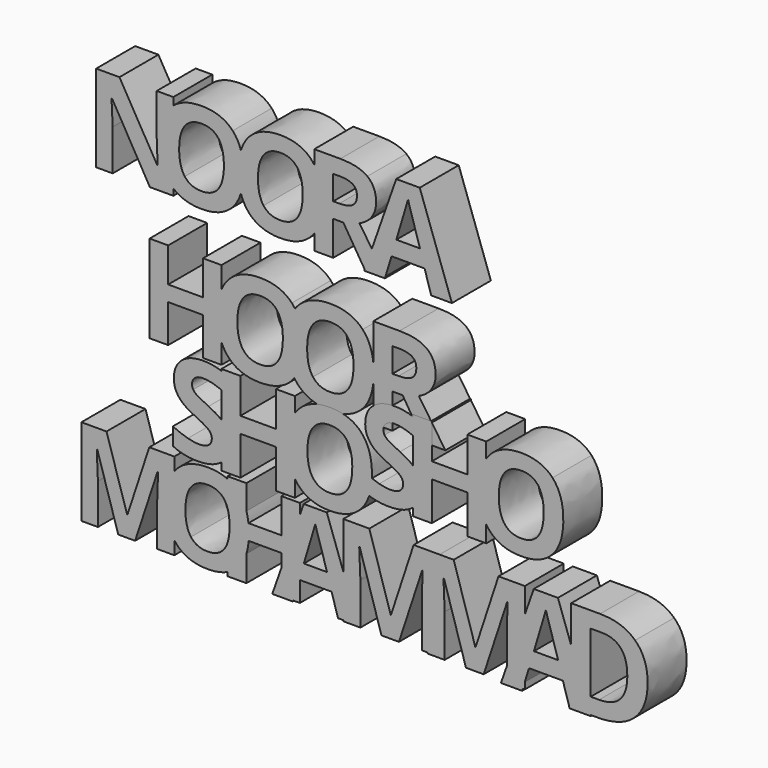
from build123d import *

# Parameters (mm, degrees)
F4_DEPTH = 25
F5_DEPTH = 25
F6_DEPTH = 25
F2_W     = 6.2625637302
F2_H     = 46.2371155878


with BuildPart() as f4:
    # F0 (on Front) → F4 (new body)
    with BuildSketch(Plane.XZ):
        with BuildLine():
            Line((-21.3353137972, -33.1943402998), (-11.8071950997, -33.1943402998))
            Line((-11.8071950997, -33.1943402998), (-11.8071950997, -23.0057868832))
            add(Edge.make_bspline(
                [(-11.8071950997, -23.0057868832), (-13.9013277173, -17.99866493), (-13.9013277173, -11.0128203345)],
                knots=[0.3919372789, 0.3919372789, 0.3919372789, 1, 1, 1], degree=2))
            add(Edge.make_bspline(
                [(-13.9013277173, -11.0128203345), (-13.9013277173, -4.036271611), (-11.8071950997, 0.9371130219)],
                knots=[0, 0, 0, 0.6072535887, 0.6072535887, 0.6072535887], degree=2))
            Line((-11.8071950997, 0.9371130219), (-11.8071950997, 11.8718857132))
            Line((-11.8071950997, 11.8718857132), (-21.3353137972, 11.8718857132))
            Line((-21.3353137972, 11.8718857132), (-21.3353137972, -5.793601437))
            Line((-21.3353137972, -5.793601437), (-39.1783435318, -5.793601437))
            Line((-39.1783435318, -5.793601437), (-39.1783435318, 11.8718857132))
            Line((-39.1783435318, 11.8718857132), (-48.73605266, 11.8718857132))
            Line((-48.73605266, 11.8718857132), (-48.73605266, -33.1943402998))
            Line((-48.73605266, -33.1943402998), (-39.1783435318, -33.1943402998))
            Line((-39.1783435318, -33.1943402998), (-39.1783435318, -13.7435638284))
            Line((-39.1783435318, -13.7435638284), (-21.3353137972, -13.7435638284))
            Line((-21.3353137972, -13.7435638284), (-21.3353137972, -33.1943402998))
        make_face()
        with BuildLine():
            add(Edge.make_bspline(
                [(-11.8071950997, -23.0057868832), (-13.9013277173, -17.99866493), (-13.9013277173, -11.0128203345)],
                knots=[0.3919372789, 0.3919372789, 0.3919372789, 1, 1, 1], degree=2))
            Line((-11.8071950997, -23.0057868832), (-11.8071950997, 0.9371130219))
            add(Edge.make_bspline(
                [(-13.9013277173, -11.0128203345), (-13.9013277173, -4.036271611), (-11.8071950997, 0.9371130219)],
                knots=[0, 0, 0, 0.6072535887, 0.6072535887, 0.6072535887], degree=2))
        make_face()
        with BuildLine():
            Line((-11.8071950997, 0.9371130219), (-11.8071950997, -23.0057868832))
            add(Edge.make_bspline(
                [(-8.237534045, -28.6385462427), (-10.457385925, -26.2332134056), (-11.8071950997, -23.0057868832)],
                knots=[0, 0, 0, 0.3919372789, 0.3919372789, 0.3919372789], degree=2))
            add(Edge.make_bspline(
                [(7.9986744822, -34.7755813418), (-2.5737403727, -34.7755813418), (-8.237534045, -28.6385462427)],
                knots=[0, 0, 0, 1, 1, 1], degree=2))
            add(Edge.make_bspline(
                [(24.2348830094, -28.6385462427), (18.5710893372, -34.7755813418), (7.9986744822, -34.7755813418)],
                knots=[0, 0, 0, 1, 1, 1], degree=2))
            add(Edge.make_bspline(
                [(25.5832055823, -26.9929228199), (24.9547978497, -27.858478518), (24.2348830094, -28.6385462427)],
                knots=[0.8728917609, 0.8728917609, 0.8728917609, 1, 1, 1], degree=2))
            add(Edge.make_bspline(
                [(25.5832055823, -26.9929228199), (21.7115614933, -21.0599088889), (21.7115614933, -11.4686214765)],
                knots=[0.1811928258, 0.1811928258, 0.1811928258, 1, 1, 1], degree=2))
            add(Edge.make_bspline(
                [(21.7115614933, -11.4686214765), (21.7115614933, -1.5095593905), (25.8969432134, 4.4459327701)],
                knots=[0, 0, 0, 0.8502040585, 0.8502040585, 0.8502040585], degree=2))
            add(Edge.make_bspline(
                [(24.2801933588, 6.4820090087), (25.1569815466, 5.5290125286), (25.8969432134, 4.4459327701)],
                knots=[0, 0, 0, 0.1560542476, 0.1560542476, 0.1560542476], degree=2))
            add(Edge.make_bspline(
                [(8.0590882814, 12.5888372083), (18.6617100359, 12.5888372083), (24.2801933588, 6.4820090087)],
                knots=[0, 0, 0, 1, 1, 1], degree=2))
            add(Edge.make_bspline(
                [(-8.2224305952, 6.5323538414), (-2.5435334731, 12.5888372083), (8.0590882814, 12.5888372083)],
                knots=[0, 0, 0, 1, 1, 1], degree=2))
            add(Edge.make_bspline(
                [(-11.8071950997, 0.9371130219), (-10.4527970599, 4.1536917341), (-8.2224305952, 6.5323538414)],
                knots=[0.6072535887, 0.6072535887, 0.6072535887, 1, 1, 1], degree=2))
        make_face()
        with BuildLine():
            add(Edge.make_bspline(
                [(-3.6712577243, -11.0732341337), (-3.6712577243, -18.7860624946), (-0.7462229478, -22.6877870243)],
                knots=[0, 0, 0, 1, 1, 1], degree=2))
            add(Edge.make_bspline(
                [(-0.7160160482, 0.5463532402), (-3.6712577243, -3.3704747394), (-3.6712577243, -11.0732341337)],
                knots=[0, 0, 0, 1, 1, 1], degree=2))
            add(Edge.make_bspline(
                [(8.0590882814, 4.4631812198), (2.2392256279, 4.4631812198), (-0.7160160482, 0.5463532402)],
                knots=[0, 0, 0, 1, 1, 1], degree=2))
            add(Edge.make_bspline(
                [(19.6686066888, -11.0732341337), (19.6686066888, 4.4631812198), (8.0590882814, 4.4631812198)],
                knots=[0, 0, 0, 1, 1, 1], degree=2))
            add(Edge.make_bspline(
                [(7.9986744822, -26.5895115541), (19.6686066888, -26.5895115541), (19.6686066888, -11.0732341337)],
                knots=[0, 0, 0, 1, 1, 1], degree=2))
            add(Edge.make_bspline(
                [(-0.7462229478, -22.6877870243), (2.1788118287, -26.5895115541), (7.9986744822, -26.5895115541)],
                knots=[0, 0, 0, 1, 1, 1], degree=2))
        make_face(mode=Mode.SUBTRACT)
        with BuildLine():
            add(Edge.make_bspline(
                [(25.5832055823, -26.9929228199), (21.7115614933, -21.0599088889), (21.7115614933, -11.4686214765)],
                knots=[0.1811928258, 0.1811928258, 0.1811928258, 1, 1, 1], degree=2))
            add(Edge.make_bspline(
                [(29.8986766817, -11.0732341337), (29.8986766817, -21.048882977), (25.5832055823, -26.9929228199)],
                knots=[0, 0, 0, 0.8728917609, 0.8728917609, 0.8728917609], degree=2))
            add(Edge.make_bspline(
                [(25.8969432134, 4.4459327701), (29.8986766817, -1.4113929713), (29.8986766817, -11.0732341337)],
                knots=[0.1560542476, 0.1560542476, 0.1560542476, 1, 1, 1], degree=2))
            add(Edge.make_bspline(
                [(21.7115614933, -11.4686214765), (21.7115614933, -1.5095593905), (25.8969432134, 4.4459327701)],
                knots=[0, 0, 0, 0.8502040585, 0.8502040585, 0.8502040585], degree=2))
        make_face()
        with BuildLine():
            add(Edge.make_bspline(
                [(29.8986766817, -11.0732341337), (29.8986766817, -21.048882977), (25.5832055823, -26.9929228199)],
                knots=[0, 0, 0, 0.8728917609, 0.8728917609, 0.8728917609], degree=2))
            add(Edge.make_bspline(
                [(27.4862976764, -29.4396004781), (26.4399569092, -28.3058321268), (25.5832055823, -26.9929228199)],
                knots=[0, 0, 0, 0.1811928258, 0.1811928258, 0.1811928258], degree=2))
            add(Edge.make_bspline(
                [(44.0405414011, -35.6968479511), (33.2610338594, -35.6968479511), (27.4862976764, -29.4396004781)],
                knots=[0, 0, 0, 1, 1, 1], degree=2))
            add(Edge.make_bspline(
                [(60.5947851258, -29.4396004781), (54.8200489428, -35.6968479511), (44.0405414011, -35.6968479511)],
                knots=[0, 0, 0, 1, 1, 1], degree=2))
            add(Edge.make_bspline(
                [(66.087589583, -16.4160509741), (65.0935584026, -24.5649297009), (60.5947851258, -29.4396004781)],
                knots=[0.2209560516, 0.2209560516, 0.2209560516, 1, 1, 1], degree=2))
            Line((66.087589583, -16.4160509741), (66.087589583, -6.6192053935))
            add(Edge.make_bspline(
                [(60.6409830153, 6.3688969555), (65.0986725029, 1.5237559622), (66.087589583, -6.6192053935)],
                knots=[0, 0, 0, 0.7781547856, 0.7781547856, 0.7781547856], degree=2))
            add(Edge.make_bspline(
                [(44.102138587, 12.5953458356), (54.9124447217, 12.5953458356), (60.6409830153, 6.3688969555)],
                knots=[0, 0, 0, 1, 1, 1], degree=2))
            add(Edge.make_bspline(
                [(27.5016969728, 6.4202279438), (33.2918324524, 12.5953458356), (44.102138587, 12.5953458356)],
                knots=[0, 0, 0, 1, 1, 1], degree=2))
            add(Edge.make_bspline(
                [(25.8969432134, 4.4459327701), (26.6343581774, 5.4952203455), (27.5016969728, 6.4202279438)],
                knots=[0.8502040585, 0.8502040585, 0.8502040585, 1, 1, 1], degree=2))
            add(Edge.make_bspline(
                [(25.8969432134, 4.4459327701), (29.8986766817, -1.4113929713), (29.8986766817, -11.0732341337)],
                knots=[0.1560542476, 0.1560542476, 0.1560542476, 1, 1, 1], degree=2))
        make_face()
        with BuildLine():
            add(Edge.make_bspline(
                [(32.1420183146, -11.5302186625), (32.1420183146, -19.3941260691), (35.1243487345, -23.3722776618)],
                knots=[0, 0, 0, 1, 1, 1], degree=2))
            add(Edge.make_bspline(
                [(35.1551473274, 0.3169734357), (32.1420183146, -3.6765774535), (32.1420183146, -11.5302186625)],
                knots=[0, 0, 0, 1, 1, 1], degree=2))
            add(Edge.make_bspline(
                [(44.102138587, 4.310524325), (38.1682763403, 4.310524325), (35.1551473274, 0.3169734357)],
                knots=[0, 0, 0, 1, 1, 1], degree=2))
            add(Edge.make_bspline(
                [(55.9390644876, -11.5302186625), (55.9390644876, 4.310524325), (44.102138587, 4.310524325)],
                knots=[0, 0, 0, 1, 1, 1], degree=2))
            add(Edge.make_bspline(
                [(44.0405414011, -27.3504292546), (55.9390644876, -27.3504292546), (55.9390644876, -11.5302186625)],
                knots=[0, 0, 0, 1, 1, 1], degree=2))
            add(Edge.make_bspline(
                [(35.1243487345, -23.3722776618), (38.1066791543, -27.3504292546), (44.0405414011, -27.3504292546)],
                knots=[0, 0, 0, 1, 1, 1], degree=2))
        make_face(mode=Mode.SUBTRACT)
        with BuildLine():
            Line((66.087589583, -6.6192053935), (66.087589583, -16.4160509741))
            add(Edge.make_bspline(
                [(66.3695213088, -11.5302186625), (66.3695213088, -14.10482826), (66.087589583, -16.4160509741)],
                knots=[0, 0, 0, 0.2209560516, 0.2209560516, 0.2209560516], degree=2))
            add(Edge.make_bspline(
                [(66.087589583, -6.6192053935), (66.3695213088, -8.9406934074), (66.3695213088, -11.5302186625)],
                knots=[0.7781547856, 0.7781547856, 0.7781547856, 1, 1, 1], degree=2))
        make_face()
        with BuildLine():
            add(Edge.make_bspline(
                [(66.3695213088, -11.5302186625), (66.3695213088, -14.10482826), (66.087589583, -16.4160509741)],
                knots=[0, 0, 0, 0.2209560516, 0.2209560516, 0.2209560516], degree=2))
            Line((66.087589583, -16.4160509741), (66.087589583, -34.4568653964))
            Line((66.087589583, -34.4568653964), (75.9107906423, -34.4568653964))
            Line((75.9107906423, -34.4568653964), (75.9107906423, -16.6858938206))
            Line((75.9107906423, -16.6858938206), (81.131583775, -16.6858938206))
            Line((81.131583775, -16.6858938206), (92.1915552462, -34.4568653964))
            Line((92.1915552462, -34.4568653964), (103.0893273192, -34.4568653964))
            add(Edge.make_bspline(
                [(89.4645778624, -14.2731777709), (99.9264390525, -29.8950073193), (103.0893273192, -34.4568653964)],
                knots=[0, 0, 0, 1, 1, 1], degree=2))
            add(Edge.make_bspline(
                [(95.8359729767, -9.2855462733), (93.5905250565, -12.4687094649), (89.4645778624, -14.2731777709)],
                knots=[0, 0, 0, 1, 1, 1], degree=2))
            add(Edge.make_bspline(
                [(98.0814208969, -2.0169857372), (98.0814208969, -6.1023830818), (95.8359729767, -9.2855462733)],
                knots=[0, 0, 0, 1, 1, 1], degree=2))
            add(Edge.make_bspline(
                [(93.5550439382, 8.4246005281), (98.0814208969, 4.9880007767), (98.0814208969, -2.0169857372)],
                knots=[0, 0, 0, 1, 1, 1], degree=2))
            add(Edge.make_bspline(
                [(79.5805520288, 11.8612002795), (89.0286669795, 11.8612002795), (93.5550439382, 8.4246005281)],
                knots=[0, 0, 0, 1, 1, 1], degree=2))
            Line((79.5805520288, 11.8612002795), (66.087589583, 11.8612002795))
            Line((66.087589583, 11.8612002795), (66.087589583, -6.6192053935))
            add(Edge.make_bspline(
                [(66.087589583, -6.6192053935), (66.3695213088, -8.9406934074), (66.3695213088, -11.5302186625)],
                knots=[0.7781547856, 0.7781547856, 0.7781547856, 1, 1, 1], degree=2))
        make_face()
        with BuildLine():
            Line((79.0736789091, -8.6975734545), (75.9107906423, -8.6975734545))
            Line((75.9107906423, -8.6975734545), (75.9107906423, 3.8120551391))
            Line((75.9107906423, 3.8120551391), (78.891204586, 3.8120551391))
            add(Edge.make_bspline(
                [(85.9012598311, 2.4181540599), (83.6355369861, 3.8120551391), (78.891204586, 3.8120551391)],
                knots=[0, 0, 0, 1, 1, 1], degree=2))
            add(Edge.make_bspline(
                [(88.166982676, -2.270422297), (88.166982676, 1.0242529808), (85.9012598311, 2.4181540599)],
                knots=[0, 0, 0, 1, 1, 1], degree=2))
            add(Edge.make_bspline(
                [(85.9519471431, -7.1465417083), (88.166982676, -5.5955099621), (88.166982676, -2.270422297)],
                knots=[0, 0, 0, 1, 1, 1], degree=2))
            add(Edge.make_bspline(
                [(79.0736789091, -8.6975734545), (83.7369116101, -8.6975734545), (85.9519471431, -7.1465417083)],
                knots=[0, 0, 0, 1, 1, 1], degree=2))
        make_face(mode=Mode.SUBTRACT)
    extrude(amount=F4_DEPTH)


with BuildPart() as f5:
    # F1 (on Front) → F5 (new body)
    with BuildSketch(Plane.XZ):
        with BuildLine():
            Line((-48.5764728851, 35.1428589012), (-36.5549885101, 35.1428589012))
            Line((-36.5549885101, 35.1428589012), (-36.5549885101, 38.4932039616))
            add(Edge.make_bspline(
                [(-36.5549885101, 38.4932039616), (-37.337133854, 39.1602999713), (-38.0419799443, 39.9240398682)],
                knots=[0.8734596848, 0.8734596848, 0.8734596848, 1, 1, 1], degree=2))
            add(Edge.make_bspline(
                [(-38.0419799443, 39.9240398682), (-43.6121106118, 45.9595858982), (-43.6121106118, 57.2582865055)],
                knots=[0, 0, 0, 1, 1, 1], degree=2))
            add(Edge.make_bspline(
                [(-43.6121106118, 57.2582865055), (-43.6121106118, 68.5569871128), (-38.0271262626, 74.5133135066)],
                knots=[0, 0, 0, 1, 1, 1], degree=2))
            add(Edge.make_bspline(
                [(-38.0271262626, 74.5133135066), (-37.328899138, 75.257965307), (-36.5549885101, 75.9095217551)],
                knots=[0, 0, 0, 0.1250186358, 0.1250186358, 0.1250186358], degree=2))
            Line((-36.5549885101, 75.9095217551), (-36.5549885101, 79.7619995262))
            Line((-36.5549885101, 79.7619995262), (-45.0706135101, 79.7619995262))
            Line((-45.0706135101, 79.7619995262), (-45.0706135101, 58.6389526512))
            add(Edge.make_bspline(
                [(-44.6116291351, 46.3440307762), (-45.0706135101, 55.0452026512), (-45.0706135101, 58.6389526512)],
                knots=[0, 0, 0, 1, 1, 1], degree=2))
            Line((-44.6116291351, 46.3440307762), (-44.8264728851, 46.3440307762))
            Line((-44.8264728851, 46.3440307762), (-64.2014728851, 79.7619995262))
            Line((-64.2014728851, 79.7619995262), (-76.1350666351, 79.7619995262))
            Line((-76.1350666351, 79.7619995262), (-76.1350666351, 35.1428589012))
            Line((-76.1350666351, 35.1428589012), (-67.6780353851, 35.1428589012))
            Line((-67.6780353851, 35.1428589012), (-67.6780353851, 56.1389526512))
            add(Edge.make_bspline(
                [(-68.2639728851, 68.8928589012), (-67.6780353851, 59.9573120262), (-67.6780353851, 56.1389526512)],
                knots=[0, 0, 0, 1, 1, 1], degree=2))
            Line((-68.2639728851, 68.8928589012), (-67.9905353851, 68.8928589012))
            Line((-67.9905353851, 68.8928589012), (-48.5764728851, 35.1428589012))
        make_face()
        with BuildLine():
            add(Edge.make_bspline(
                [(-36.5549885101, 38.4932039616), (-37.337133854, 39.1602999713), (-38.0419799443, 39.9240398682)],
                knots=[0.8734596848, 0.8734596848, 0.8734596848, 1, 1, 1], degree=2))
            Line((-36.5549885101, 38.4932039616), (-36.5549885101, 75.9095217551))
            add(Edge.make_bspline(
                [(-38.0271262626, 74.5133135066), (-37.328899138, 75.257965307), (-36.5549885101, 75.9095217551)],
                knots=[0, 0, 0, 0.1250186358, 0.1250186358, 0.1250186358], degree=2))
            add(Edge.make_bspline(
                [(-43.6121106118, 57.2582865055), (-43.6121106118, 68.5569871128), (-38.0271262626, 74.5133135066)],
                knots=[0, 0, 0, 1, 1, 1], degree=2))
            add(Edge.make_bspline(
                [(-38.0419799443, 39.9240398682), (-43.6121106118, 45.9595858982), (-43.6121106118, 57.2582865055)],
                knots=[0, 0, 0, 1, 1, 1], degree=2))
        make_face()
        with BuildLine():
            Line((-36.5549885101, 75.9095217551), (-36.5549885101, 38.4932039616))
            add(Edge.make_bspline(
                [(-22.0742720308, 33.8884938383), (-31.1561365749, 33.8884938383), (-36.5549885101, 38.4932039616)],
                knots=[0, 0, 0, 0.8734596848, 0.8734596848, 0.8734596848], degree=2))
            add(Edge.make_bspline(
                [(-6.1065641174, 39.9240398682), (-11.6766947848, 33.8884938383), (-22.0742720308, 33.8884938383)],
                knots=[0, 0, 0, 1, 1, 1], degree=2))
            add(Edge.make_bspline(
                [(-1.8486114519, 47.5145455032), (-3.2399502207, 43.0301752816), (-6.1065641174, 39.9240398682)],
                knots=[0.4853596679, 0.4853596679, 0.4853596679, 1, 1, 1], degree=2))
            add(Edge.make_bspline(
                [(-1.8486114519, 47.5145455032), (-3.1656606093, 51.7641834469), (-3.1656606093, 57.2582865055)],
                knots=[0.5137402743, 0.5137402743, 0.5137402743, 1, 1, 1], degree=2))
            add(Edge.make_bspline(
                [(-3.1656606093, 57.2582865055), (-3.1656606093, 62.729767225), (-1.8559519315, 66.94843264)],
                knots=[0, 0, 0, 0.4842575186, 0.4842575186, 0.4842575186], degree=2))
            add(Edge.make_bspline(
                [(-6.062003072, 74.463801234), (-3.2366355234, 71.3928596243), (-1.8559519315, 66.94843264)],
                knots=[0, 0, 0, 0.5113260246, 0.5113260246, 0.5113260246], degree=2))
            add(Edge.make_bspline(
                [(-22.0148573037, 80.4696399004), (-11.5875726942, 80.4696399004), (-6.062003072, 74.463801234)],
                knots=[0, 0, 0, 1, 1, 1], degree=2))
            add(Edge.make_bspline(
                [(-36.5549885101, 75.9095217551), (-31.1385370158, 80.4696399004), (-22.0148573037, 80.4696399004)],
                knots=[0.1250186358, 0.1250186358, 0.1250186358, 1, 1, 1], degree=2))
        make_face()
        with BuildLine():
            add(Edge.make_bspline(
                [(-33.5512168195, 57.1988717784), (-33.5512168195, 49.6135916161), (-30.6745537815, 45.7763904896)],
                knots=[0, 0, 0, 1, 1, 1], degree=2))
            add(Edge.make_bspline(
                [(-30.6448464179, 68.6263042945), (-33.5512168195, 64.7742494862), (-33.5512168195, 57.1988717784)],
                knots=[0, 0, 0, 1, 1, 1], degree=2))
            add(Edge.make_bspline(
                [(-22.0148573037, 72.4783591027), (-27.7384760163, 72.4783591027), (-30.6448464179, 68.6263042945)],
                knots=[0, 0, 0, 1, 1, 1], degree=2))
            add(Edge.make_bspline(
                [(-10.5973272422, 57.1988717784), (-10.5973272422, 72.4783591027), (-22.0148573037, 72.4783591027)],
                knots=[0, 0, 0, 1, 1, 1], degree=2))
            add(Edge.make_bspline(
                [(-22.0742720308, 41.9391893631), (-10.5973272422, 41.9391893631), (-10.5973272422, 57.1988717784)],
                knots=[0, 0, 0, 1, 1, 1], degree=2))
            add(Edge.make_bspline(
                [(-30.6745537815, 45.7763904896), (-27.7978907434, 41.9391893631), (-22.0742720308, 41.9391893631)],
                knots=[0, 0, 0, 1, 1, 1], degree=2))
        make_face(mode=Mode.SUBTRACT)
        with BuildLine():
            add(Edge.make_bspline(
                [(-1.8486114519, 47.5145455032), (-3.1656606093, 51.7641834469), (-3.1656606093, 57.2582865055)],
                knots=[0.5137402743, 0.5137402743, 0.5137402743, 1, 1, 1], degree=2))
            add(Edge.make_bspline(
                [(-0.5364334499, 57.1988717784), (-0.5364334499, 51.7437757163), (-1.8486114519, 47.5145455032)],
                knots=[0, 0, 0, 0.4853596679, 0.4853596679, 0.4853596679], degree=2))
            add(Edge.make_bspline(
                [(-1.8559519315, 66.94843264), (-0.5364334499, 62.7008964337), (-0.5364334499, 57.1988717784)],
                knots=[0.5113260246, 0.5113260246, 0.5113260246, 1, 1, 1], degree=2))
            add(Edge.make_bspline(
                [(-3.1656606093, 57.2582865055), (-3.1656606093, 62.729767225), (-1.8559519315, 66.94843264)],
                knots=[0, 0, 0, 0.4842575186, 0.4842575186, 0.4842575186], degree=2))
        make_face()
        with BuildLine():
            add(Edge.make_bspline(
                [(-0.5364334499, 57.1988717784), (-0.5364334499, 51.7437757163), (-1.8486114519, 47.5145455032)],
                knots=[0, 0, 0, 0.4853596679, 0.4853596679, 0.4853596679], degree=2))
            add(Edge.make_bspline(
                [(2.4044700582, 39.9240398682), (-0.4571303986, 43.0247429409), (-1.8486114519, 47.5145455032)],
                knots=[0, 0, 0, 0.5137402743, 0.5137402743, 0.5137402743], degree=2))
            add(Edge.make_bspline(
                [(18.3721779716, 33.8884938383), (7.9746007256, 33.8884938383), (2.4044700582, 39.9240398682)],
                knots=[0, 0, 0, 1, 1, 1], degree=2))
            add(Edge.make_bspline(
                [(34.3398858851, 39.9240398682), (28.7697552176, 33.8884938383), (18.3721779716, 33.8884938383)],
                knots=[0, 0, 0, 1, 1, 1], degree=2))
            add(Edge.make_bspline(
                [(35.7973932629, 41.7259413865), (35.1238020662, 40.7734566014), (34.3398858851, 39.9240398682)],
                knots=[0.8592643103, 0.8592643103, 0.8592643103, 1, 1, 1], degree=2))
            Line((35.7973932629, 41.7259413865), (35.7973932629, 72.7158650742))
            add(Edge.make_bspline(
                [(34.3844469305, 74.463801234), (35.1429853678, 73.6393324845), (35.7973932629, 72.7158650742)],
                knots=[0, 0, 0, 0.1372778716, 0.1372778716, 0.1372778716], degree=2))
            add(Edge.make_bspline(
                [(18.4315926988, 80.4696399004), (28.8588773083, 80.4696399004), (34.3844469305, 74.463801234)],
                knots=[0, 0, 0, 1, 1, 1], degree=2))
            add(Edge.make_bspline(
                [(2.4193237399, 74.5133135066), (8.0043080892, 80.4696399004), (18.4315926988, 80.4696399004)],
                knots=[0, 0, 0, 1, 1, 1], degree=2))
            add(Edge.make_bspline(
                [(-1.8559519315, 66.94843264), (-0.461089947, 71.4413829522), (2.4193237399, 74.5133135066)],
                knots=[0.4842575186, 0.4842575186, 0.4842575186, 1, 1, 1], degree=2))
            add(Edge.make_bspline(
                [(-1.8559519315, 66.94843264), (-0.5364334499, 62.7008964337), (-0.5364334499, 57.1988717784)],
                knots=[0.5113260246, 0.5113260246, 0.5113260246, 1, 1, 1], degree=2))
        make_face()
        with BuildLine():
            add(Edge.make_bspline(
                [(6.895233183, 57.1988717784), (6.895233183, 49.6135916161), (9.771896221, 45.7763904896)],
                knots=[0, 0, 0, 1, 1, 1], degree=2))
            add(Edge.make_bspline(
                [(9.8016035846, 68.6263042945), (6.895233183, 64.7742494862), (6.895233183, 57.1988717784)],
                knots=[0, 0, 0, 1, 1, 1], degree=2))
            add(Edge.make_bspline(
                [(18.4315926988, 72.4783591027), (12.7079739862, 72.4783591027), (9.8016035846, 68.6263042945)],
                knots=[0, 0, 0, 1, 1, 1], degree=2))
            add(Edge.make_bspline(
                [(29.8491227603, 57.1988717784), (29.8491227603, 72.4783591027), (18.4315926988, 72.4783591027)],
                knots=[0, 0, 0, 1, 1, 1], degree=2))
            add(Edge.make_bspline(
                [(18.3721779716, 41.9391893631), (29.8491227603, 41.9391893631), (29.8491227603, 57.1988717784)],
                knots=[0, 0, 0, 1, 1, 1], degree=2))
            add(Edge.make_bspline(
                [(9.771896221, 45.7763904896), (12.6485592591, 41.9391893631), (18.3721779716, 41.9391893631)],
                knots=[0, 0, 0, 1, 1, 1], degree=2))
        make_face(mode=Mode.SUBTRACT)
        with BuildLine():
            Line((35.7973932629, 72.7158650742), (35.7973932629, 41.7259413865))
            add(Edge.make_bspline(
                [(39.9100165526, 57.1988717784), (39.9100165526, 47.541354548), (35.7973932629, 41.7259413865)],
                knots=[0, 0, 0, 0.8592643103, 0.8592643103, 0.8592643103], degree=2))
            add(Edge.make_bspline(
                [(35.7973932629, 72.7158650742), (39.9100165526, 66.9123385475), (39.9100165526, 57.1988717784)],
                knots=[0.1372778716, 0.1372778716, 0.1372778716, 1, 1, 1], degree=2))
        make_face()
        with BuildLine():
            add(Edge.make_bspline(
                [(39.9100165526, 57.1988717784), (39.9100165526, 47.541354548), (35.7973932629, 41.7259413865)],
                knots=[0, 0, 0, 0.8592643103, 0.8592643103, 0.8592643103], degree=2))
            Line((35.7973932629, 41.7259413865), (35.7973932629, 33.8131673634))
            Line((35.7973932629, 33.8131673634), (45.5399000121, 33.8131673634))
            Line((45.5399000121, 33.8131673634), (45.5399000121, 51.4381563534))
            Line((45.5399000121, 51.4381563534), (50.7178060759, 51.4381563534))
            Line((50.7178060759, 51.4381563534), (61.6644474176, 33.8492816769))
            Line((61.6644474176, 33.8492816769), (65.3522718239, 44.3388900938))
            add(Edge.make_bspline(
                [(58.9823474049, 53.8310527479), (62.6096596302, 48.4146882719), (65.3522718239, 44.3388900938)],
                knots=[0, 0, 0, 0.3495894388, 0.3495894388, 0.3495894388], degree=2))
            add(Edge.make_bspline(
                [(65.30140364, 58.7777125215), (63.0744013233, 55.6206979505), (58.9823474049, 53.8310527479)],
                knots=[0, 0, 0, 1, 1, 1], degree=2))
            add(Edge.make_bspline(
                [(67.5284059568, 65.9865642647), (67.5284059568, 61.9347270924), (65.30140364, 58.7777125215)],
                knots=[0, 0, 0, 1, 1, 1], degree=2))
            add(Edge.make_bspline(
                [(63.0392116704, 76.3423763923), (67.5284059568, 72.934007158), (67.5284059568, 65.9865642647)],
                knots=[0, 0, 0, 1, 1, 1], degree=2))
            add(Edge.make_bspline(
                [(49.1795155365, 79.7507456265), (58.550017384, 79.7507456265), (63.0392116704, 76.3423763923)],
                knots=[0, 0, 0, 1, 1, 1], degree=2))
            Line((49.1795155365, 79.7507456265), (35.7973932629, 79.7507456265))
            Line((35.7973932629, 79.7507456265), (35.7973932629, 72.7158650742))
            add(Edge.make_bspline(
                [(35.7973932629, 72.7158650742), (39.9100165526, 66.9123385475), (39.9100165526, 57.1988717784)],
                knots=[0.1372778716, 0.1372778716, 0.1372778716, 1, 1, 1], degree=2))
        make_face()
        with BuildLine():
            Line((48.6768062099, 59.3608553403), (45.5399000121, 59.3608553403))
            Line((45.5399000121, 59.3608553403), (45.5399000121, 71.7677215204))
            Line((45.5399000121, 71.7677215204), (48.4958308524, 71.7677215204))
            add(Edge.make_bspline(
                [(55.448300839, 70.3852708723), (53.2011901492, 71.7677215204), (48.4958308524, 71.7677215204)],
                knots=[0, 0, 0, 1, 1, 1], degree=2))
            add(Edge.make_bspline(
                [(57.6954115288, 65.7352096014), (57.6954115288, 69.0028202242), (55.448300839, 70.3852708723)],
                knots=[0, 0, 0, 1, 1, 1], degree=2))
            add(Edge.make_bspline(
                [(55.4985717717, 60.8991458796), (57.6954115288, 62.437436419), (57.6954115288, 65.7352096014)],
                knots=[0, 0, 0, 1, 1, 1], degree=2))
            add(Edge.make_bspline(
                [(48.6768062099, 59.3608553403), (53.3017320145, 59.3608553403), (55.4985717717, 60.8991458796)],
                knots=[0, 0, 0, 1, 1, 1], degree=2))
        make_face(mode=Mode.SUBTRACT)
        with BuildLine():
            Line((65.3522718239, 44.3388900938), (61.6644474176, 33.8492816769))
            Line((61.6644474176, 33.8492816769), (61.6869235819, 33.8131673634))
            Line((61.6869235819, 33.8131673634), (72.2655823064, 33.8131673634))
            Line((72.2655823064, 33.8131673634), (72.33566955, 34.0435447683))
            add(Edge.make_bspline(
                [(65.3522718239, 44.3388900938), (70.260972013, 37.0440668107), (72.33566955, 34.0435447683)],
                knots=[0.3495894388, 0.3495894388, 0.3495894388, 0.9752811602, 0.9752811602, 0.9752811602], degree=2))
        make_face()
        Polygon((61.6869235819, 33.8131673634), (61.6644474176, 33.8492816769), (61.421725899, 33.1588871777), (72.0665319926, 33.1588871777), (72.2655823064, 33.8131673634), align=None)
        with BuildLine():
            Line((77.8681552371, 79.9389354128), (65.3522718239, 44.3388900938))
            add(Edge.make_bspline(
                [(65.3522718239, 44.3388900938), (70.260972013, 37.0440668107), (72.33566955, 34.0435447683)],
                knots=[0.3495894388, 0.3495894388, 0.3495894388, 0.9752811602, 0.9752811602, 0.9752811602], degree=2))
            Line((72.33566955, 34.0435447683), (75.4414657253, 44.2523249458))
            Line((75.4414657253, 44.2523249458), (92.4282923077, 44.2523249458))
            Line((92.4282923077, 44.2523249458), (95.8032260404, 33.1588871777))
            Line((95.8032260404, 33.1588871777), (106.448032134, 33.1588871777))
            Line((106.448032134, 33.1588871777), (89.9404257494, 79.9389354128))
            Line((89.9404257494, 79.9389354128), (77.8681552371, 79.9389354128))
        make_face()
        with BuildLine():
            add(Edge.make_bspline(
                [(90.0627798424, 52.5316185741), (85.382735784, 67.6015643656), (84.7913576677, 69.579622203)],
                knots=[0, 0, 0, 1, 1, 1], degree=2))
            Line((90.0627798424, 52.5316185741), (77.9293322836, 52.5316185741))
            add(Edge.make_bspline(
                [(83.9450751909, 72.6996515752), (82.8948692257, 68.6211818076), (77.9293322836, 52.5316185741)],
                knots=[0, 0, 0, 1, 1, 1], degree=2))
            add(Edge.make_bspline(
                [(84.7913576677, 69.579622203), (84.1999795514, 71.5576800403), (83.9450751909, 72.6996515752)],
                knots=[0, 0, 0, 1, 1, 1], degree=2))
        make_face(mode=Mode.SUBTRACT)
        with BuildLine():
            Line((72.33566955, 34.0435447683), (72.2655823064, 33.8131673634))
            Line((72.2655823064, 33.8131673634), (72.4951741034, 33.8131673634))
            add(Edge.make_bspline(
                [(72.33566955, 34.0435447683), (72.4176334217, 33.925004885), (72.4951741034, 33.8131673634)],
                knots=[0.9752811602, 0.9752811602, 0.9752811602, 1, 1, 1], degree=2))
        make_face()
    extrude(amount=F5_DEPTH)


with BuildPart() as f6:
    # F3 (on Front) → F6 (new body)
    with BuildSketch(Plane.XZ):
        with BuildLine():
            add(Edge.make_bspline(
                [(-9.773376744, -60.1399672845), (-7.4308009773, -63.172986435), (-7.4308009773, -67.5819606149)],
                knots=[0, 0, 0, 1, 1, 1], degree=2))
            add(Edge.make_bspline(
                [(-7.4308009773, -67.5819606149), (-7.4308009773, -73.6874528237), (-11.8249799418, -77.203782343)],
                knots=[0, 0, 0, 1, 1, 1], degree=2))
            add(Edge.make_bspline(
                [(-11.8249799418, -77.203782343), (-11.8411305754, -77.2167064752), (-11.857327512, -77.2295831053)],
                knots=[0, 0, 0, 0.003675461, 0.003675461, 0.003675461], degree=2))
            Line((-11.857327512, -77.2295831053), (-11.857327512, -81.0456089675))
            Line((-11.857327512, -81.0456089675), (-2.1004989459, -81.0456089675))
            Line((-2.1004989459, -81.0456089675), (-2.1004989459, -61.1896069733))
            Line((-2.1004989459, -61.1896069733), (16.1142615042, -61.1896069733))
            Line((16.1142615042, -61.1896069733), (16.1142615042, -81.0456089675))
            Line((16.1142615042, -81.0456089675), (25.8408831707, -81.0456089675))
            Line((25.8408831707, -81.0456089675), (25.8408831707, -72.4579250864))
            add(Edge.make_bspline(
                [(25.8408831707, -72.4579250864), (22.1995292231, -66.7496005995), (22.1995292231, -57.600601227)],
                knots=[0.1926675383, 0.1926675383, 0.1926675383, 1, 1, 1], degree=2))
            add(Edge.make_bspline(
                [(22.1995292231, -57.600601227), (22.1995292231, -48.4637761771), (25.8408831707, -42.8101256923)],
                knots=[0, 0, 0, 0.8062581665, 0.8062581665, 0.8062581665], degree=2))
            Line((25.8408831707, -42.8101256923), (25.8408831707, -35.0405008988))
            Line((25.8408831707, -35.0405008988), (16.1142615042, -35.0405008988))
            Line((16.1142615042, -35.0405008988), (16.1142615042, -53.0740199514))
            Line((16.1142615042, -53.0740199514), (-2.1004989459, -53.0740199514))
            Line((-2.1004989459, -53.0740199514), (-2.1004989459, -35.0405008988))
            Line((-2.1004989459, -35.0405008988), (-11.857327512, -35.0405008988))
            Line((-11.857327512, -35.0405008988), (-11.857327512, -35.9465561363))
            add(Edge.make_bspline(
                [(-11.857327512, -35.9465561363), (-9.8085950891, -36.6209872168), (-7.6477974694, -37.5575368934)],
                knots=[0.3794034527, 0.3794034527, 0.3794034527, 1, 1, 1], degree=2))
            Line((-7.6477974694, -37.5575368934), (-10.7252022661, -44.9945984854))
            add(Edge.make_bspline(
                [(-10.7252022661, -44.9945984854), (-11.3075641299, -44.7559255904), (-11.857327512, -44.5404823221)],
                knots=[0, 0, 0, 0.1613176213, 0.1613176213, 0.1613176213], degree=2))
            Line((-11.857327512, -44.5404823221), (-11.857327512, -58.0527789062))
            add(Edge.make_bspline(
                [(-11.857327512, -58.0527789062), (-10.5796303791, -59.096080999), (-9.773376744, -60.1399672845)],
                knots=[0.6558260157, 0.6558260157, 0.6558260157, 1, 1, 1], degree=2))
        make_face()
        with BuildLine():
            add(Edge.make_bspline(
                [(-7.4308009773, -67.5819606149), (-7.4308009773, -73.6874528237), (-11.8249799418, -77.203782343)],
                knots=[0, 0, 0, 1, 1, 1], degree=2))
            add(Edge.make_bspline(
                [(-9.773376744, -60.1399672845), (-7.4308009773, -63.172986435), (-7.4308009773, -67.5819606149)],
                knots=[0, 0, 0, 1, 1, 1], degree=2))
            add(Edge.make_bspline(
                [(-11.857327512, -58.0527789062), (-10.5796303791, -59.096080999), (-9.773376744, -60.1399672845)],
                knots=[0.6558260157, 0.6558260157, 0.6558260157, 1, 1, 1], degree=2))
            Line((-11.857327512, -58.0527789062), (-11.857327512, -77.2295831053))
            add(Edge.make_bspline(
                [(-11.8249799418, -77.203782343), (-11.8411305754, -77.2167064752), (-11.857327512, -77.2295831053)],
                knots=[0, 0, 0, 0.003675461, 0.003675461, 0.003675461], degree=2))
        make_face()
        with BuildLine():
            add(Edge.make_bspline(
                [(-11.857327512, -77.2295831053), (-16.2479073967, -80.7201118623), (-24.0408960979, -80.7201118623)],
                knots=[0.003675461, 0.003675461, 0.003675461, 1, 1, 1], degree=2))
            Line((-11.857327512, -77.2295831053), (-11.857327512, -58.0527789062))
            add(Edge.make_bspline(
                [(-18.4384412116, -54.0788607218), (-14.2919886375, -56.0647592245), (-11.857327512, -58.0527789062)],
                knots=[0, 0, 0, 0.6558260157, 0.6558260157, 0.6558260157], degree=2))
            add(Edge.make_bspline(
                [(-24.4896842974, -50.9225481098), (-23.2123640372, -51.800397555), (-18.4384412116, -54.0788607218)],
                knots=[0, 0, 0, 1, 1, 1], degree=2))
            add(Edge.make_bspline(
                [(-26.3538814339, -49.1027366194), (-25.7670045576, -50.0446986646), (-24.4896842974, -50.9225481098)],
                knots=[0, 0, 0, 1, 1, 1], degree=2))
            add(Edge.make_bspline(
                [(-26.9407583101, -46.8982495295), (-26.9407583101, -48.1607745743), (-26.3538814339, -49.1027366194)],
                knots=[0, 0, 0, 1, 1, 1], degree=2))
            add(Edge.make_bspline(
                [(-25.490827204, -43.6038482407), (-26.9407583101, -44.8663732855), (-26.9407583101, -46.8982495295)],
                knots=[0, 0, 0, 1, 1, 1], degree=2))
            add(Edge.make_bspline(
                [(-21.328439947, -42.3413231959), (-24.0408960979, -42.3413231959), (-25.490827204, -43.6038482407)],
                knots=[0, 0, 0, 1, 1, 1], degree=2))
            add(Edge.make_bspline(
                [(-16.6926057981, -42.9282000722), (-19.0499767802, -42.3413231959), (-21.328439947, -42.3413231959)],
                knots=[0, 0, 0, 1, 1, 1], degree=2))
            add(Edge.make_bspline(
                [(-11.857327512, -44.5404823221), (-14.7155202954, -43.4204033668), (-16.6926057981, -42.9282000722)],
                knots=[0.1613176213, 0.1613176213, 0.1613176213, 1, 1, 1], degree=2))
            Line((-11.857327512, -44.5404823221), (-11.857327512, -35.9465561363))
            add(Edge.make_bspline(
                [(-14.3204396006, -35.2198928651), (-13.1098258676, -35.5342407896), (-11.857327512, -35.9465561363)],
                knots=[0, 0, 0, 0.3794034527, 0.3794034527, 0.3794034527], degree=2))
            add(Edge.make_bspline(
                [(-21.0226721627, -34.3913608045), (-17.5112743818, -34.3913608045), (-14.3204396006, -35.2198928651)],
                knots=[0, 0, 0, 1, 1, 1], degree=2))
            add(Edge.make_bspline(
                [(-32.2275819352, -37.8090555546), (-28.1736929242, -34.3913608045), (-21.0226721627, -34.3913608045)],
                knots=[0, 0, 0, 1, 1, 1], degree=2))
            add(Edge.make_bspline(
                [(-36.2814709463, -47.2138807907), (-36.2814709463, -41.2267503048), (-32.2275819352, -37.8090555546)],
                knots=[0, 0, 0, 1, 1, 1], degree=2))
            add(Edge.make_bspline(
                [(-35.0485363322, -52.7571548155), (-36.2814709463, -50.3800568796), (-36.2814709463, -47.2138807907)],
                knots=[0, 0, 0, 1, 1, 1], degree=2))
            add(Edge.make_bspline(
                [(-31.749203305, -56.9195420725), (-33.8156017181, -55.1342527514), (-35.0485363322, -52.7571548155)],
                knots=[0, 0, 0, 1, 1, 1], degree=2))
            add(Edge.make_bspline(
                [(-25.5598715424, -60.6479363455), (-29.6828048918, -58.7048313937), (-31.749203305, -56.9195420725)],
                knots=[0, 0, 0, 1, 1, 1], degree=2))
            add(Edge.make_bspline(
                [(-19.7157614718, -63.7006824499), (-21.1508973625, -62.7488569278), (-25.5598715424, -60.6479363455)],
                knots=[0, 0, 0, 1, 1, 1], degree=2))
            add(Edge.make_bspline(
                [(-17.5408648126, -65.6881730477), (-18.280625581, -64.6525079719), (-19.7157614718, -63.7006824499)],
                knots=[0, 0, 0, 1, 1, 1], degree=2))
            add(Edge.make_bspline(
                [(-16.8011040441, -68.0455440298), (-16.8011040441, -66.7238381235), (-17.5408648126, -65.6881730477)],
                knots=[0, 0, 0, 1, 1, 1], degree=2))
            add(Edge.make_bspline(
                [(-18.4828268577, -71.6210544106), (-16.8011040441, -70.4226419657), (-16.8011040441, -68.0455440298)],
                knots=[0, 0, 0, 1, 1, 1], degree=2))
            add(Edge.make_bspline(
                [(-23.3011353294, -72.8194668554), (-20.1645496713, -72.8194668554), (-18.4828268577, -71.6210544106)],
                knots=[0, 0, 0, 1, 1, 1], degree=2))
            add(Edge.make_bspline(
                [(-29.0860645386, -71.9909347948), (-25.9248201882, -72.8194668554), (-23.3011353294, -72.8194668554)],
                knots=[0, 0, 0, 1, 1, 1], degree=2))
            add(Edge.make_bspline(
                [(-36.8042352226, -69.1206630133), (-32.2473088891, -71.1624027341), (-29.0860645386, -71.9909347948)],
                knots=[0, 0, 0, 1, 1, 1], degree=2))
            Line((-36.8042352226, -69.1206630133), (-36.8042352226, -77.9977922345))
            add(Edge.make_bspline(
                [(-24.0408960979, -80.7201118623), (-31.2609611978, -80.7201118623), (-36.8042352226, -77.9977922345)],
                knots=[0, 0, 0, 1, 1, 1], degree=2))
        make_face()
        with BuildLine():
            Line((-11.857327512, -35.9465561363), (-11.857327512, -44.5404823221))
            add(Edge.make_bspline(
                [(-10.7252022661, -44.9945984854), (-11.3075641299, -44.7559255904), (-11.857327512, -44.5404823221)],
                knots=[0, 0, 0, 0.1613176213, 0.1613176213, 0.1613176213], degree=2))
            Line((-10.7252022661, -44.9945984854), (-7.6477974694, -37.5575368934))
            add(Edge.make_bspline(
                [(-11.857327512, -35.9465561363), (-9.8085950891, -36.6209872168), (-7.6477974694, -37.5575368934)],
                knots=[0.3794034527, 0.3794034527, 0.3794034527, 1, 1, 1], degree=2))
        make_face()
        with BuildLine():
            add(Edge.make_bspline(
                [(25.8408831707, -72.4579250864), (22.1995292231, -66.7496005995), (22.1995292231, -57.600601227)],
                knots=[0.1926675383, 0.1926675383, 0.1926675383, 1, 1, 1], degree=2))
            Line((25.8408831707, -72.4579250864), (25.8408831707, -42.8101256923))
            add(Edge.make_bspline(
                [(22.1995292231, -57.600601227), (22.1995292231, -48.4637761771), (25.8408831707, -42.8101256923)],
                knots=[0, 0, 0, 0.8062581665, 0.8062581665, 0.8062581665], degree=2))
        make_face()
        with BuildLine():
            Line((25.8408831707, -42.8101256923), (25.8408831707, -72.4579250864))
            add(Edge.make_bspline(
                [(27.7862641378, -74.9865202815), (26.7098816745, -73.8202000835), (25.8408831707, -72.4579250864)],
                knots=[0, 0, 0, 0.1926675383, 0.1926675383, 0.1926675383], degree=2))
            add(Edge.make_bspline(
                [(43.8015708933, -81.0400579358), (33.3729990525, -81.0400579358), (27.7862641378, -74.9865202815)],
                knots=[0, 0, 0, 1, 1, 1], degree=2))
            add(Edge.make_bspline(
                [(59.8168776487, -74.9865202815), (54.230142734, -81.0400579358), (43.8015708933, -81.0400579358)],
                knots=[0, 0, 0, 1, 1, 1], degree=2))
            add(Edge.make_bspline(
                [(63.9854978765, -67.6943049535), (62.5888957332, -71.982884686), (59.8168776487, -74.9865202815)],
                knots=[0.5038214401, 0.5038214401, 0.5038214401, 1, 1, 1], degree=2))
            add(Edge.make_bspline(
                [(63.9854978765, -67.6943049535), (62.6635387575, -67.2220253013), (61.4252531353, -66.6138992662)],
                knots=[0.7766147557, 0.7766147557, 0.7766147557, 1, 1, 1], degree=2))
            Line((61.4252531353, -66.6138992662), (61.4252531353, -57.736770045))
            add(Edge.make_bspline(
                [(61.4252531353, -57.736770045), (63.5492553917, -58.6884333936), (65.3700414458, -59.3765236477)],
                knots=[0, 0, 0, 0.4661041458, 0.4661041458, 0.4661041458], degree=2))
            add(Edge.make_bspline(
                [(65.4036125634, -57.6601930661), (65.4036125634, -58.5340397989), (65.3700414458, -59.3765236477)],
                knots=[0, 0, 0, 0.0775182334, 0.0775182334, 0.0775182334], degree=2))
            add(Edge.make_bspline(
                [(59.861571528, -40.3437978239), (65.4036125634, -46.3675395586), (65.4036125634, -57.6601930661)],
                knots=[0, 0, 0, 1, 1, 1], degree=2))
            add(Edge.make_bspline(
                [(43.8611627324, -34.3200560892), (54.3195304926, -34.3200560892), (59.861571528, -40.3437978239)],
                knots=[0, 0, 0, 1, 1, 1], degree=2))
            add(Edge.make_bspline(
                [(27.8011620976, -40.294137958), (33.4027949721, -34.3200560892), (43.8611627324, -34.3200560892)],
                knots=[0, 0, 0, 1, 1, 1], degree=2))
            add(Edge.make_bspline(
                [(25.8408831707, -42.8101256923), (26.7158914739, -41.4515675327), (27.8011620976, -40.294137958)],
                knots=[0.8062581665, 0.8062581665, 0.8062581665, 1, 1, 1], degree=2))
        make_face()
        with BuildLine():
            add(Edge.make_bspline(
                [(32.2904139757, -57.6601930661), (32.2904139757, -65.2680845233), (35.175652185, -69.1167241312)],
                knots=[0, 0, 0, 1, 1, 1], degree=2))
            add(Edge.make_bspline(
                [(35.2054481045, -46.1986960145), (32.2904139757, -50.0622335821), (32.2904139757, -57.6601930661)],
                knots=[0, 0, 0, 1, 1, 1], degree=2))
            add(Edge.make_bspline(
                [(43.8611627324, -42.3351584468), (38.1204822334, -42.3351584468), (35.2054481045, -46.1986960145)],
                knots=[0, 0, 0, 1, 1, 1], degree=2))
            add(Edge.make_bspline(
                [(55.3127278108, -57.6601930661), (55.3127278108, -42.3351584468), (43.8611627324, -42.3351584468)],
                knots=[0, 0, 0, 1, 1, 1], degree=2))
            add(Edge.make_bspline(
                [(43.8015708933, -72.9653637391), (55.3127278108, -72.9653637391), (55.3127278108, -57.6601930661)],
                knots=[0, 0, 0, 1, 1, 1], degree=2))
            add(Edge.make_bspline(
                [(35.175652185, -69.1167241312), (38.0608903943, -72.9653637391), (43.8015708933, -72.9653637391)],
                knots=[0, 0, 0, 1, 1, 1], degree=2))
        make_face(mode=Mode.SUBTRACT)
        with BuildLine():
            add(Edge.make_bspline(
                [(63.9854978765, -67.6943049535), (62.6635387575, -67.2220253013), (61.4252531353, -66.6138992662)],
                knots=[0.7766147557, 0.7766147557, 0.7766147557, 1, 1, 1], degree=2))
            add(Edge.make_bspline(
                [(65.3700414458, -59.3765236477), (65.185420687, -64.0096731701), (63.9854978765, -67.6943049535)],
                knots=[0.0775182334, 0.0775182334, 0.0775182334, 0.5038214401, 0.5038214401, 0.5038214401], degree=2))
            add(Edge.make_bspline(
                [(61.4252531353, -57.736770045), (63.5492553917, -58.6884333936), (65.3700414458, -59.3765236477)],
                knots=[0, 0, 0, 0.4661041458, 0.4661041458, 0.4661041458], degree=2))
            Line((61.4252531353, -57.736770045), (61.4252531353, -66.6138992662))
        make_face()
        with BuildLine():
            add(Edge.make_bspline(
                [(65.3700414458, -59.3765236477), (65.185420687, -64.0096731701), (63.9854978765, -67.6943049535)],
                knots=[0.0775182334, 0.0775182334, 0.0775182334, 0.5038214401, 0.5038214401, 0.5038214401], degree=2))
            add(Edge.make_bspline(
                [(74.18859226, -69.336218894), (68.5813831663, -69.336218894), (63.9854978765, -67.6943049535)],
                knots=[0, 0, 0, 0.7766147557, 0.7766147557, 0.7766147557], degree=2))
            add(Edge.make_bspline(
                [(86.3721608459, -65.845690137), (81.9815809612, -69.336218894), (74.18859226, -69.336218894)],
                knots=[0.003675461, 0.003675461, 0.003675461, 1, 1, 1], degree=2))
            Line((86.3721608459, -65.845690137), (86.3721608459, -46.6688859379))
            add(Edge.make_bspline(
                [(79.7910471463, -42.6949677535), (83.9374997204, -44.6808662562), (86.3721608459, -46.6688859379)],
                knots=[0, 0, 0, 0.6558260157, 0.6558260157, 0.6558260157], degree=2))
            add(Edge.make_bspline(
                [(73.7398040605, -39.5386551415), (75.0171243207, -40.4165045867), (79.7910471463, -42.6949677535)],
                knots=[0, 0, 0, 1, 1, 1], degree=2))
            add(Edge.make_bspline(
                [(71.875606924, -37.7188436511), (72.4624838003, -38.6608056963), (73.7398040605, -39.5386551415)],
                knots=[0, 0, 0, 1, 1, 1], degree=2))
            add(Edge.make_bspline(
                [(71.2887300478, -35.5143565612), (71.2887300478, -36.776881606), (71.875606924, -37.7188436511)],
                knots=[0, 0, 0, 1, 1, 1], degree=2))
            add(Edge.make_bspline(
                [(72.7386611539, -32.2199552724), (71.2887300478, -33.4824803172), (71.2887300478, -35.5143565612)],
                knots=[0, 0, 0, 1, 1, 1], degree=2))
            add(Edge.make_bspline(
                [(76.9010484109, -30.9574302276), (74.18859226, -30.9574302276), (72.7386611539, -32.2199552724)],
                knots=[0, 0, 0, 1, 1, 1], degree=2))
            add(Edge.make_bspline(
                [(81.5368825598, -31.5443071039), (79.1795115777, -30.9574302276), (76.9010484109, -30.9574302276)],
                knots=[0, 0, 0, 1, 1, 1], degree=2))
            add(Edge.make_bspline(
                [(86.3721608459, -33.1565893538), (83.5139680625, -32.0365103985), (81.5368825598, -31.5443071039)],
                knots=[0.1613176213, 0.1613176213, 0.1613176213, 1, 1, 1], degree=2))
            Line((86.3721608459, -33.1565893538), (86.3721608459, -24.562663168))
            add(Edge.make_bspline(
                [(83.9090487573, -23.8359998968), (85.1196624903, -24.1503478213), (86.3721608459, -24.562663168)],
                knots=[0, 0, 0, 0.3794034527, 0.3794034527, 0.3794034527], degree=2))
            add(Edge.make_bspline(
                [(77.2068161952, -23.0074678362), (80.7182139761, -23.0074678362), (83.9090487573, -23.8359998968)],
                knots=[0, 0, 0, 1, 1, 1], degree=2))
            add(Edge.make_bspline(
                [(66.0019064227, -26.4251625863), (70.0557954337, -23.0074678362), (77.2068161952, -23.0074678362)],
                knots=[0, 0, 0, 1, 1, 1], degree=2))
            add(Edge.make_bspline(
                [(61.9480174116, -35.8299878224), (61.9480174116, -29.8428573365), (66.0019064227, -26.4251625863)],
                knots=[0, 0, 0, 1, 1, 1], degree=2))
            add(Edge.make_bspline(
                [(63.1809520257, -41.3732618472), (61.9480174116, -38.9961639113), (61.9480174116, -35.8299878224)],
                knots=[0, 0, 0, 1, 1, 1], degree=2))
            add(Edge.make_bspline(
                [(66.4802850529, -45.5356491042), (64.4138866398, -43.7503597831), (63.1809520257, -41.3732618472)],
                knots=[0, 0, 0, 1, 1, 1], degree=2))
            add(Edge.make_bspline(
                [(72.6696168155, -49.2640433772), (68.5466834661, -47.3209384254), (66.4802850529, -45.5356491042)],
                knots=[0, 0, 0, 1, 1, 1], degree=2))
            add(Edge.make_bspline(
                [(78.5137268861, -52.3167894816), (77.0785909954, -51.3649639595), (72.6696168155, -49.2640433772)],
                knots=[0, 0, 0, 1, 1, 1], degree=2))
            add(Edge.make_bspline(
                [(80.6886235453, -54.3042800794), (79.9488627769, -53.2686150036), (78.5137268861, -52.3167894816)],
                knots=[0, 0, 0, 1, 1, 1], degree=2))
            add(Edge.make_bspline(
                [(81.4283843138, -56.6616510615), (81.4283843138, -55.3399451552), (80.6886235453, -54.3042800794)],
                knots=[0, 0, 0, 1, 1, 1], degree=2))
            add(Edge.make_bspline(
                [(79.7466615002, -60.2371614423), (81.4283843138, -59.0387489974), (81.4283843138, -56.6616510615)],
                knots=[0, 0, 0, 1, 1, 1], degree=2))
            add(Edge.make_bspline(
                [(74.9283530285, -61.4355738871), (78.0649386866, -61.4355738871), (79.7466615002, -60.2371614423)],
                knots=[0, 0, 0, 1, 1, 1], degree=2))
            add(Edge.make_bspline(
                [(69.1434238193, -60.6070418265), (72.3046681697, -61.4355738871), (74.9283530285, -61.4355738871)],
                knots=[0, 0, 0, 1, 1, 1], degree=2))
            add(Edge.make_bspline(
                [(65.3700414458, -59.3765236477), (67.4556485666, -60.1646919943), (69.1434238193, -60.6070418265)],
                knots=[0.4661041458, 0.4661041458, 0.4661041458, 1, 1, 1], degree=2))
        make_face()
        with BuildLine():
            Line((86.3721608459, -46.6688859379), (86.3721608459, -65.845690137))
            add(Edge.make_bspline(
                [(86.4045084161, -65.8198893747), (86.3883577825, -65.8328135069), (86.3721608459, -65.845690137)],
                knots=[0, 0, 0, 0.003675461, 0.003675461, 0.003675461], degree=2))
            add(Edge.make_bspline(
                [(90.7986873806, -56.1980676466), (90.7986873806, -62.3035598554), (86.4045084161, -65.8198893747)],
                knots=[0, 0, 0, 1, 1, 1], degree=2))
            add(Edge.make_bspline(
                [(88.4561116139, -48.7560743162), (90.7986873806, -51.7890934667), (90.7986873806, -56.1980676466)],
                knots=[0, 0, 0, 1, 1, 1], degree=2))
            add(Edge.make_bspline(
                [(86.3721608459, -46.6688859379), (87.6498579788, -47.7121880307), (88.4561116139, -48.7560743162)],
                knots=[0.6558260157, 0.6558260157, 0.6558260157, 1, 1, 1], degree=2))
        make_face()
        with BuildLine():
            add(Edge.make_bspline(
                [(86.4045084161, -65.8198893747), (86.3883577825, -65.8328135069), (86.3721608459, -65.845690137)],
                knots=[0, 0, 0, 0.003675461, 0.003675461, 0.003675461], degree=2))
            Line((86.3721608459, -65.845690137), (86.3721608459, -69.6617159992))
            Line((86.3721608459, -69.6617159992), (96.128989412, -69.6617159992))
            Line((96.128989412, -69.6617159992), (96.128989412, -49.805714005))
            Line((96.128989412, -49.805714005), (114.3437498621, -49.805714005))
            Line((114.3437498621, -49.805714005), (114.3437498621, -69.6617159992))
            Line((114.3437498621, -69.6617159992), (124.0703715286, -69.6617159992))
            Line((124.0703715286, -69.6617159992), (124.0703715286, -61.0740321181))
            add(Edge.make_bspline(
                [(124.0703715286, -61.0740321181), (120.429017581, -55.3657076312), (120.429017581, -46.2167082587)],
                knots=[0.1926675383, 0.1926675383, 0.1926675383, 1, 1, 1], degree=2))
            add(Edge.make_bspline(
                [(120.429017581, -46.2167082587), (120.429017581, -37.0798832088), (124.0703715286, -31.426232724)],
                knots=[0, 0, 0, 0.8062581665, 0.8062581665, 0.8062581665], degree=2))
            Line((124.0703715286, -31.426232724), (124.0703715286, -23.6566079305))
            Line((124.0703715286, -23.6566079305), (114.3437498621, -23.6566079305))
            Line((114.3437498621, -23.6566079305), (114.3437498621, -41.6901269831))
            Line((114.3437498621, -41.6901269831), (96.128989412, -41.6901269831))
            Line((96.128989412, -41.6901269831), (96.128989412, -23.6566079305))
            Line((96.128989412, -23.6566079305), (86.3721608459, -23.6566079305))
            Line((86.3721608459, -23.6566079305), (86.3721608459, -24.562663168))
            add(Edge.make_bspline(
                [(86.3721608459, -24.562663168), (88.4208932688, -25.2370942485), (90.5816908885, -26.1736439251)],
                knots=[0.3794034527, 0.3794034527, 0.3794034527, 1, 1, 1], degree=2))
            Line((90.5816908885, -26.1736439251), (87.5042860918, -33.6107055171))
            add(Edge.make_bspline(
                [(87.5042860918, -33.6107055171), (86.9219242281, -33.3720326221), (86.3721608459, -33.1565893538)],
                knots=[0, 0, 0, 0.1613176213, 0.1613176213, 0.1613176213], degree=2))
            Line((86.3721608459, -33.1565893538), (86.3721608459, -46.6688859379))
            add(Edge.make_bspline(
                [(86.3721608459, -46.6688859379), (87.6498579788, -47.7121880307), (88.4561116139, -48.7560743162)],
                knots=[0.6558260157, 0.6558260157, 0.6558260157, 1, 1, 1], degree=2))
            add(Edge.make_bspline(
                [(88.4561116139, -48.7560743162), (90.7986873806, -51.7890934667), (90.7986873806, -56.1980676466)],
                knots=[0, 0, 0, 1, 1, 1], degree=2))
            add(Edge.make_bspline(
                [(90.7986873806, -56.1980676466), (90.7986873806, -62.3035598554), (86.4045084161, -65.8198893747)],
                knots=[0, 0, 0, 1, 1, 1], degree=2))
        make_face()
        with BuildLine():
            Line((86.3721608459, -24.562663168), (86.3721608459, -33.1565893538))
            add(Edge.make_bspline(
                [(87.5042860918, -33.6107055171), (86.9219242281, -33.3720326221), (86.3721608459, -33.1565893538)],
                knots=[0, 0, 0, 0.1613176213, 0.1613176213, 0.1613176213], degree=2))
            Line((87.5042860918, -33.6107055171), (90.5816908885, -26.1736439251))
            add(Edge.make_bspline(
                [(86.3721608459, -24.562663168), (88.4208932688, -25.2370942485), (90.5816908885, -26.1736439251)],
                knots=[0.3794034527, 0.3794034527, 0.3794034527, 1, 1, 1], degree=2))
        make_face()
        with BuildLine():
            add(Edge.make_bspline(
                [(124.0703715286, -61.0740321181), (120.429017581, -55.3657076312), (120.429017581, -46.2167082587)],
                knots=[0.1926675383, 0.1926675383, 0.1926675383, 1, 1, 1], degree=2))
            Line((124.0703715286, -61.0740321181), (124.0703715286, -31.426232724))
            add(Edge.make_bspline(
                [(120.429017581, -46.2167082587), (120.429017581, -37.0798832088), (124.0703715286, -31.426232724)],
                knots=[0, 0, 0, 0.8062581665, 0.8062581665, 0.8062581665], degree=2))
        make_face()
        with BuildLine():
            Line((124.0703715286, -31.426232724), (124.0703715286, -61.0740321181))
            add(Edge.make_bspline(
                [(126.0157524957, -63.6026273132), (124.9393700324, -62.4363071152), (124.0703715286, -61.0740321181)],
                knots=[0, 0, 0, 0.1926675383, 0.1926675383, 0.1926675383], degree=2))
            add(Edge.make_bspline(
                [(142.0310592512, -69.6561649675), (131.6024874104, -69.6561649675), (126.0157524957, -63.6026273132)],
                knots=[0, 0, 0, 1, 1, 1], degree=2))
            add(Edge.make_bspline(
                [(158.0463660066, -63.6026273132), (152.4596310919, -69.6561649675), (142.0310592512, -69.6561649675)],
                knots=[0, 0, 0, 1, 1, 1], degree=2))
            add(Edge.make_bspline(
                [(163.6331009213, -46.2763000978), (163.6331009213, -57.549089659), (158.0463660066, -63.6026273132)],
                knots=[0, 0, 0, 1, 1, 1], degree=2))
            add(Edge.make_bspline(
                [(158.0910598859, -28.9599048556), (163.6331009213, -34.9836465903), (163.6331009213, -46.2763000978)],
                knots=[0, 0, 0, 1, 1, 1], degree=2))
            add(Edge.make_bspline(
                [(142.0906510903, -22.9361631209), (152.5490188506, -22.9361631209), (158.0910598859, -28.9599048556)],
                knots=[0, 0, 0, 1, 1, 1], degree=2))
            add(Edge.make_bspline(
                [(126.0306504555, -28.9102449897), (131.63228333, -22.9361631209), (142.0906510903, -22.9361631209)],
                knots=[0, 0, 0, 1, 1, 1], degree=2))
            add(Edge.make_bspline(
                [(124.0703715286, -31.426232724), (124.9453798318, -30.0676745644), (126.0306504555, -28.9102449897)],
                knots=[0.8062581665, 0.8062581665, 0.8062581665, 1, 1, 1], degree=2))
        make_face()
        with BuildLine():
            add(Edge.make_bspline(
                [(130.5199023336, -46.2763000978), (130.5199023336, -53.884191555), (133.4051405429, -57.7328311629)],
                knots=[0, 0, 0, 1, 1, 1], degree=2))
            add(Edge.make_bspline(
                [(133.4349364624, -34.8148030462), (130.5199023336, -38.6783406138), (130.5199023336, -46.2763000978)],
                knots=[0, 0, 0, 1, 1, 1], degree=2))
            add(Edge.make_bspline(
                [(142.0906510903, -30.9512654785), (136.3499705913, -30.9512654785), (133.4349364624, -34.8148030462)],
                knots=[0, 0, 0, 1, 1, 1], degree=2))
            add(Edge.make_bspline(
                [(153.5422161687, -46.2763000978), (153.5422161687, -30.9512654785), (142.0906510903, -30.9512654785)],
                knots=[0, 0, 0, 1, 1, 1], degree=2))
            add(Edge.make_bspline(
                [(142.0310592512, -61.5814707708), (153.5422161687, -61.5814707708), (153.5422161687, -46.2763000978)],
                knots=[0, 0, 0, 1, 1, 1], degree=2))
            add(Edge.make_bspline(
                [(133.4051405429, -57.7328311629), (136.2903787522, -61.5814707708), (142.0310592512, -61.5814707708)],
                knots=[0, 0, 0, 1, 1, 1], degree=2))
        make_face(mode=Mode.SUBTRACT)
    extrude(amount=F6_DEPTH)


with BuildPart() as f6b:
    # F2 (on Front) → F6, piece 2 (new body)
    with BuildSketch(Plane.XZ):
        with BuildLine():
            Line((-75.5733697707, -92.1196341246), (-64.8311822707, -127.1196341246))
            Line((-64.8311822707, -127.1196341246), (-56.1593072707, -127.1196341246))
            Line((-56.1593072707, -127.1196341246), (-44.6554010207, -92.1782278746))
            Line((-44.6554010207, -92.1782278746), (-44.3819635207, -92.1782278746))
            add(Edge.make_bspline(
                [(-44.7921197707, -102.5493216246), (-44.7432916457, -100.5961966246), (-44.3819635207, -92.1782278746)],
                knots=[0, 0, 0, 1, 1, 1], degree=2))
            add(Edge.make_bspline(
                [(-44.8409478957, -105.9965872496), (-44.8409478957, -104.5024466246), (-44.7921197707, -102.5493216246)],
                knots=[0, 0, 0, 1, 1, 1], degree=2))
            Line((-44.8409478957, -105.9965872496), (-44.8409478957, -127.1196341246))
            Line((-44.8409478957, -127.1196341246), (-36.0225885207, -127.1196341246))
            Line((-36.0225885207, -127.1196341246), (-36.0225885207, -120.3385569702))
            add(Edge.make_bspline(
                [(-36.0225885207, -120.3385569702), (-40.2785209824, -114.5436056064), (-40.2785209824, -104.7272709476)],
                knots=[0.1205553949, 0.1205553949, 0.1205553949, 1, 1, 1], degree=2))
            add(Edge.make_bspline(
                [(-40.2785209824, -104.7272709476), (-40.2785209824, -94.9239986162), (-36.0225885207, -89.1917822477)],
                knots=[0, 0, 0, 0.8782743523, 0.8782743523, 0.8782743523], degree=2))
            Line((-36.0225885207, -89.1917822477), (-36.0225885207, -82.5004934996))
            Line((-36.0225885207, -82.5004934996), (-48.8936822707, -82.5004934996))
            Line((-48.8936822707, -82.5004934996), (-60.0948541457, -116.6215872496))
            Line((-60.0948541457, -116.6215872496), (-60.2804010207, -116.6215872496))
            Line((-60.2804010207, -116.6215872496), (-70.8370416457, -82.5004934996))
            Line((-70.8370416457, -82.5004934996), (-83.7179010207, -82.5004934996))
            Line((-83.7179010207, -82.5004934996), (-83.7179010207, -127.1196341246))
            Line((-83.7179010207, -127.1196341246), (-75.2608697707, -127.1196341246))
            Line((-75.2608697707, -127.1196341246), (-75.2608697707, -106.3676809996))
            add(Edge.make_bspline(
                [(-75.8468072707, -92.1196341246), (-75.2608697707, -102.7934622496), (-75.2608697707, -106.3676809996)],
                knots=[0, 0, 0, 1, 1, 1], degree=2))
            Line((-75.8468072707, -92.1196341246), (-75.5733697707, -92.1196341246))
        make_face()
        with BuildLine():
            add(Edge.make_bspline(
                [(-36.0225885207, -120.3385569702), (-40.2785209824, -114.5436056064), (-40.2785209824, -104.7272709476)],
                knots=[0.1205553949, 0.1205553949, 0.1205553949, 1, 1, 1], degree=2))
            Line((-36.0225885207, -120.3385569702), (-36.0225885207, -89.1917822477))
            add(Edge.make_bspline(
                [(-40.2785209824, -104.7272709476), (-40.2785209824, -94.9239986162), (-36.0225885207, -89.1917822477)],
                knots=[0, 0, 0, 0.8782743523, 0.8782743523, 0.8782743523], degree=2))
        make_face()
        with BuildLine():
            Line((-36.0225885207, -89.1917822477), (-36.0225885207, -120.3385569702))
            add(Edge.make_bspline(
                [(-34.7757967449, -121.8517487748), (-35.4391798382, -121.1329363386), (-36.0225885207, -120.3385569702)],
                knots=[0, 0, 0, 0.1205553949, 0.1205553949, 0.1205553949], degree=2))
            add(Edge.make_bspline(
                [(-19.0013205973, -127.814256193), (-29.2730725074, -127.814256193), (-34.7757967449, -121.8517487748)],
                knots=[0, 0, 0, 1, 1, 1], degree=2))
            add(Edge.make_bspline(
                [(-8.6275690506, -125.7793810251), (-13.0006616867, -127.814256193), (-19.0013205973, -127.814256193)],
                knots=[0.4158095948, 0.4158095948, 0.4158095948, 1, 1, 1], degree=2))
            Line((-8.6275690506, -125.7793810251), (-8.6275690506, -112.2966059036))
            add(Edge.make_bspline(
                [(-19.0013205973, -119.8609854284), (-10.9698257878, -119.8609854284), (-8.6275690506, -112.2966059036)],
                knots=[0, 0, 0, 0.7083660274, 0.7083660274, 0.7083660274], degree=2))
            add(Edge.make_bspline(
                [(-27.4975268201, -116.0702198425), (-24.6556754583, -119.8609854284), (-19.0013205973, -119.8609854284)],
                knots=[0, 0, 0, 1, 1, 1], degree=2))
            add(Edge.make_bspline(
                [(-30.3393781818, -104.7859666728), (-30.3393781818, -112.2794542567), (-27.4975268201, -116.0702198425)],
                knots=[0, 0, 0, 1, 1, 1], degree=2))
            add(Edge.make_bspline(
                [(-27.4681789575, -93.4968221926), (-30.3393781818, -97.3022617098), (-30.3393781818, -104.7859666728)],
                knots=[0, 0, 0, 1, 1, 1], degree=2))
            add(Edge.make_bspline(
                [(-18.9426248721, -89.6913826755), (-24.5969797331, -89.6913826755), (-27.4681789575, -93.4968221926)],
                knots=[0, 0, 0, 1, 1, 1], degree=2))
            add(Edge.make_bspline(
                [(-8.6275690506, -97.2493823934), (-10.9612558483, -89.6913826755), (-18.9426248721, -89.6913826755)],
                knots=[0.2923917928, 0.2923917928, 0.2923917928, 1, 1, 1], degree=2))
            Line((-8.6275690506, -97.2493823934), (-8.6275690506, -83.7903179984))
            add(Edge.make_bspline(
                [(-18.9426248721, -81.796807636), (-12.9715869619, -81.796807636), (-8.6275690506, -83.7903179984)],
                knots=[0, 0, 0, 0.5796505268, 0.5796505268, 0.5796505268], degree=2))
            add(Edge.make_bspline(
                [(-34.7611228136, -87.6810540874), (-29.2437246448, -81.796807636), (-18.9426248721, -81.796807636)],
                knots=[0, 0, 0, 1, 1, 1], degree=2))
            add(Edge.make_bspline(
                [(-36.0225885207, -89.1917822477), (-35.4327316792, -88.3973177978), (-34.7611228136, -87.6810540874)],
                knots=[0.8782743523, 0.8782743523, 0.8782743523, 1, 1, 1], degree=2))
        make_face()
        with BuildLine():
            Line((-8.6275690506, -112.2966059036), (-8.6275690506, -125.7793810251))
            add(Edge.make_bspline(
                [(-3.2268444498, -121.8517487748), (-5.5149299851, -124.3310165682), (-8.6275690506, -125.7793810251)],
                knots=[0, 0, 0, 0.4158095948, 0.4158095948, 0.4158095948], degree=2))
            add(Edge.make_bspline(
                [(0.9609903433, -114.4127426153), (-0.4140038557, -118.8038797222), (-3.2268444498, -121.8517487748)],
                knots=[0.4888276293, 0.4888276293, 0.4888276293, 1, 1, 1], degree=2))
            Line((0.9609903433, -114.4127426153), (0.9609903433, -108.2036821766))
            Line((0.9609903433, -108.2036821766), (2.1353291795, -108.2036821766))
            add(Edge.make_bspline(
                [(2.2758797878, -104.7859666728), (2.2758797878, -106.5604771755), (2.1353291795, -108.2036821766)],
                knots=[0, 0, 0, 0.1598186619, 0.1598186619, 0.1598186619], degree=2))
            add(Edge.make_bspline(
                [(2.0217910824, -100.2280589862), (2.2758797878, -102.3862296232), (2.2758797878, -104.7859666728)],
                knots=[0.7842514083, 0.7842514083, 0.7842514083, 1, 1, 1], degree=2))
            Line((2.0217910824, -100.2280589862), (0.9609903433, -100.2280589862))
            Line((0.9609903433, -100.2280589862), (0.9609903433, -95.1179913281))
            add(Edge.make_bspline(
                [(-3.1828226559, -87.7299671917), (-0.4032227156, -90.7511631841), (0.9609903433, -95.1179913281)],
                knots=[0, 0, 0, 0.5092052496, 0.5092052496, 0.5092052496], degree=2))
            add(Edge.make_bspline(
                [(-8.6275690506, -83.7903179984), (-5.4773853522, -85.2359666983), (-3.1828226559, -87.7299671917)],
                knots=[0.5796505268, 0.5796505268, 0.5796505268, 1, 1, 1], degree=2))
            Line((-8.6275690506, -83.7903179984), (-8.6275690506, -97.2493823934))
            add(Edge.make_bspline(
                [(-7.6632630128, -104.7859666728), (-7.6632630128, -100.3724341965), (-8.6275690506, -97.2493823934)],
                knots=[0, 0, 0, 0.2923917928, 0.2923917928, 0.2923917928], degree=2))
            add(Edge.make_bspline(
                [(-8.6275690506, -112.2966059036), (-7.6632630128, -109.1823542796), (-7.6632630128, -104.7859666728)],
                knots=[0.7083660274, 0.7083660274, 0.7083660274, 1, 1, 1], degree=2))
        make_face()
        with BuildLine():
            add(Edge.make_bspline(
                [(-3.2268444498, -121.8517487748), (-5.5149299851, -124.3310165682), (-8.6275690506, -125.7793810251)],
                knots=[0, 0, 0, 0.4158095948, 0.4158095948, 0.4158095948], degree=2))
            Line((-8.6275690506, -125.7793810251), (-8.6275690506, -127.7172416449))
            Line((-8.6275690506, -127.7172416449), (0.9609903433, -127.7172416449))
            Line((0.9609903433, -127.7172416449), (0.9609903433, -114.4127426153))
            add(Edge.make_bspline(
                [(0.9609903433, -114.4127426153), (-0.4140038557, -118.8038797222), (-3.2268444498, -121.8517487748)],
                knots=[0.4888276293, 0.4888276293, 0.4888276293, 1, 1, 1], degree=2))
        make_face()
        with BuildLine():
            Line((-8.6275690506, -82.5055513758), (-8.6275690506, -83.7903179984))
            add(Edge.make_bspline(
                [(-8.6275690506, -83.7903179984), (-5.4773853522, -85.2359666983), (-3.1828226559, -87.7299671917)],
                knots=[0.5796505268, 0.5796505268, 0.5796505268, 1, 1, 1], degree=2))
            add(Edge.make_bspline(
                [(-3.1828226559, -87.7299671917), (-0.4032227156, -90.7511631841), (0.9609903433, -95.1179913281)],
                knots=[0, 0, 0, 0.5092052496, 0.5092052496, 0.5092052496], degree=2))
            Line((0.9609903433, -95.1179913281), (0.9609903433, -82.5055513758))
            Line((0.9609903433, -82.5055513758), (-8.6275690506, -82.5055513758))
        make_face()
        with BuildLine():
            Line((0.9609903433, -108.2036821766), (0.9609903433, -114.4127426153))
            add(Edge.make_bspline(
                [(2.1353291795, -108.2036821766), (1.8459861832, -111.5864484575), (0.9609903433, -114.4127426153)],
                knots=[0.1598186619, 0.1598186619, 0.1598186619, 0.4888276293, 0.4888276293, 0.4888276293], degree=2))
            Line((2.1353291795, -108.2036821766), (0.9609903433, -108.2036821766))
        make_face()
        with BuildLine():
            add(Edge.make_bspline(
                [(0.9609903433, -95.1179913281), (1.6978671957, -97.4767244867), (2.0217910824, -100.2280589862)],
                knots=[0.5092052496, 0.5092052496, 0.5092052496, 0.7842514083, 0.7842514083, 0.7842514083], degree=2))
            Line((0.9609903433, -95.1179913281), (0.9609903433, -100.2280589862))
            Line((0.9609903433, -100.2280589862), (2.0217910824, -100.2280589862))
        make_face()
        with BuildLine():
            add(Edge.make_bspline(
                [(2.2758797878, -104.7859666728), (2.2758797878, -106.5604771755), (2.1353291795, -108.2036821766)],
                knots=[0, 0, 0, 0.1598186619, 0.1598186619, 0.1598186619], degree=2))
            Line((2.1353291795, -108.2036821766), (18.8616136081, -108.2036821766))
            Line((18.8616136081, -108.2036821766), (18.8616136081, -115.103130612))
            Line((18.8616136081, -115.103130612), (28.4204870596, -87.9139728963))
            Line((28.4204870596, -87.9139728963), (28.4204870596, -82.5055513758))
            Line((28.4204870596, -82.5055513758), (18.8616136081, -82.5055513758))
            Line((18.8616136081, -82.5055513758), (18.8616136081, -100.2280589862))
            Line((18.8616136081, -100.2280589862), (2.0217910824, -100.2280589862))
            add(Edge.make_bspline(
                [(2.0217910824, -100.2280589862), (2.2758797878, -102.3862296232), (2.2758797878, -104.7859666728)],
                knots=[0.7842514083, 0.7842514083, 0.7842514083, 1, 1, 1], degree=2))
        make_face()
        Polygon((28.4204870596, -87.9139728963), (18.8616136081, -115.103130612), (18.8616136081, -127.7172416449), (24.8506604174, -127.7172416449), (28.00532124, -117.3478429287), (28.4204870596, -117.3478429287), align=None)
        Polygon((18.8616136081, -127.7172416449), (18.8616136081, -115.103130612), (14.2443021759, -128.2365620136), (24.6926686508, -128.2365620136), (24.8506604174, -127.7172416449), align=None)
        Polygon((30.3872285399, -82.3197944019), (28.4204870596, -87.9139728963), (28.4204870596, -117.3478429287), (44.6786723388, -117.3478429287), (47.991324928, -128.2365620136), (50.7025981853, -128.2365620136), (50.7025981853, -106.3108154527), (42.2367169558, -82.3197944019), align=None)
        with BuildLine():
            add(Edge.make_bspline(
                [(42.3568131222, -109.2213356705), (37.7631347582, -94.4294911783), (37.1826699541, -92.4879364886)],
                knots=[0, 0, 0, 1, 1, 1], degree=2))
            Line((42.3568131222, -109.2213356705), (30.447276623, -109.2213356705))
            add(Edge.make_bspline(
                [(36.3520048033, -89.4254842459), (35.3211793752, -93.4286897919), (30.447276623, -109.2213356705)],
                knots=[0, 0, 0, 1, 1, 1], degree=2))
            add(Edge.make_bspline(
                [(37.1826699541, -92.4879364886), (36.6022051499, -90.5463817988), (36.3520048033, -89.4254842459)],
                knots=[0, 0, 0, 1, 1, 1], degree=2))
        make_face(mode=Mode.SUBTRACT)
        Polygon((28.00532124, -117.3478429287), (24.8506604174, -127.7172416449), (28.4204870596, -127.7172416449), (28.4204870596, -117.3478429287), align=None)
        with BuildLine():
            Line((50.7025981853, -82.5143417027), (50.7025981853, -106.3108154527))
            Line((50.7025981853, -106.3108154527), (58.4396914029, -128.2365620136))
            Line((58.4396914029, -128.2365620136), (50.7025981853, -128.2365620136))
            Line((50.7025981853, -128.2365620136), (50.7025981853, -128.7558525801))
            Line((50.7025981853, -128.7558525801), (59.46713056, -128.7558525801))
            Line((59.46713056, -128.7558525801), (59.46713056, -107.2493499286))
            add(Edge.make_bspline(
                [(58.8598881322, -92.4832382258), (59.46713056, -103.545171119), (59.46713056, -107.2493499286)],
                knots=[0, 0, 0, 1, 1, 1], degree=2))
            Line((58.8598881322, -92.4832382258), (59.1432679318, -92.4832382258))
            Line((59.1432679318, -92.4832382258), (70.2760457749, -128.7558525801))
            Line((70.2760457749, -128.7558525801), (79.2632337064, -128.7558525801))
            Line((79.2632337064, -128.7558525801), (91.1854267057, -92.5439624686))
            Line((91.1854267057, -92.5439624686), (91.4688065053, -92.5439624686))
            add(Edge.make_bspline(
                [(91.0437368059, -103.2921534408), (91.0943403415, -101.2680120148), (91.4688065053, -92.5439624686)],
                knots=[0, 0, 0, 1, 1, 1], degree=2))
            add(Edge.make_bspline(
                [(90.9931332702, -106.8647630577), (90.9931332702, -105.3162948668), (91.0437368059, -103.2921534408)],
                knots=[0, 0, 0, 1, 1, 1], degree=2))
            Line((90.9931332702, -106.8647630577), (90.9931332702, -128.7558525801))
            Line((90.9931332702, -128.7558525801), (93.8695680785, -128.7558525801))
            Line((93.8695680785, -128.7558525801), (93.8695680785, -82.5187369923))
            Line((93.8695680785, -82.5187369923), (100.1321318087, -82.5187369923))
            Line((100.1321318087, -82.5187369923), (100.1321318087, -82.5143417027))
            Line((100.1321318087, -82.5143417027), (86.7930398112, -82.5143417027))
            Line((86.7930398112, -82.5143417027), (75.184588733, -117.8760924152))
            Line((75.184588733, -117.8760924152), (74.9922952975, -117.8760924152))
            Line((74.9922952975, -117.8760924152), (64.0518108899, -82.5143417027))
            Line((64.0518108899, -82.5143417027), (50.7025981853, -82.5143417027))
        make_face()
        Polygon((58.4396914029, -128.2365620136), (50.7025981853, -106.3108154527), (50.7025981853, -128.2365620136), align=None)
        with BuildLine():
            Line((107.3674317306, -82.5187369923), (100.1321318087, -82.5187369923))
            Line((100.1321318087, -82.5187369923), (100.1321318087, -128.7558525801))
            Line((100.1321318087, -128.7558525801), (93.8695680785, -128.7558525801))
            Line((93.8695680785, -128.7558525801), (93.8695680785, -129.2751729488))
            Line((93.8695680785, -129.2751729488), (102.7316984217, -129.2751729488))
            Line((102.7316984217, -129.2751729488), (102.7316984217, -107.5291833652))
            add(Edge.make_bspline(
                [(102.1176940099, -92.5986427522), (102.7316984217, -103.7837564534), (102.7316984217, -107.5291833652)],
                knots=[0, 0, 0, 1, 1, 1], degree=2))
            Line((102.1176940099, -92.5986427522), (102.4042294021, -92.5986427522))
            Line((102.4042294021, -92.5986427522), (113.6609769513, -129.2751729488))
            Line((113.6609769513, -129.2751729488), (122.7482422455, -129.2751729488))
            Line((122.7482422455, -129.2751729488), (134.80319553, -92.6600431934))
            Line((134.80319553, -92.6600431934), (135.0897309222, -92.6600431934))
            add(Edge.make_bspline(
                [(134.6599278339, -103.5279212818), (134.7110948683, -101.4812399092), (135.0897309222, -92.6600431934)],
                knots=[0, 0, 0, 1, 1, 1], degree=2))
            add(Edge.make_bspline(
                [(134.6087607996, -107.1403139044), (134.6087607996, -105.5746026544), (134.6599278339, -103.5279212818)],
                knots=[0, 0, 0, 1, 1, 1], degree=2))
            Line((134.6087607996, -107.1403139044), (134.6087607996, -121.775115133))
            Line((134.6087607996, -121.775115133), (143.8495271968, -95.4907777304))
            Line((143.8495271968, -95.4907777304), (143.8495271968, -82.5187369923))
            Line((143.8495271968, -82.5187369923), (130.3618969515, -82.5187369923))
            Line((130.3618969515, -82.5187369923), (118.6241792798, -118.2742605712))
            Line((118.6241792798, -118.2742605712), (118.4297445494, -118.2742605712))
            Line((118.4297445494, -118.2742605712), (107.3674317306, -82.5187369923))
        make_face()
        with Locations((97.0008499436, -105.6372947862)):
            Rectangle(F2_W, F2_H)
        Polygon((148.4768711064, -82.3288100572), (143.8495271968, -95.4907777304), (143.8495271968, -125.9627177079), (145.9876775091, -118.9345982525), (163.41203269, -118.9345982525), (166.8738943737, -130.3137689829), (177.7928780525, -130.3137689829), (177.6096270603, -129.7944635153), (167.675422731, -129.7944635153), (167.675422731, -101.6424379052), (160.860086313, -82.3288100572), align=None)
        with BuildLine():
            add(Edge.make_bspline(
                [(160.9855918725, -110.4420553912), (156.1850042206, -94.9839539761), (155.5783940162, -92.9549474304)],
                knots=[0, 0, 0, 1, 1, 1], degree=2))
            Line((160.9855918725, -110.4420553912), (148.5396238861, -110.4420553912))
            add(Edge.make_bspline(
                [(154.7103138962, -89.7545556625), (153.6330578436, -93.9380743134), (148.5396238861, -110.4420553912)],
                knots=[0, 0, 0, 1, 1, 1], degree=2))
            add(Edge.make_bspline(
                [(155.5783940162, -92.9549474304), (154.9717838119, -90.9259408848), (154.7103138962, -89.7545556625)],
                knots=[0, 0, 0, 1, 1, 1], degree=2))
        make_face(mode=Mode.SUBTRACT)
        Polygon((143.8495271968, -125.9627177079), (143.8495271968, -95.4907777304), (134.6087607996, -121.775115133), (134.6087607996, -129.2751729488), (142.8417857586, -129.2751729488), align=None)
        Polygon((143.8495271968, -129.2751729488), (143.8495271968, -125.9627177079), (142.8417857586, -129.2751729488), align=None)
        Polygon((134.6087607996, -129.2751729488), (134.6087607996, -121.775115133), (131.6068321466, -130.3137689829), (142.5258158255, -130.3137689829), (142.8417857586, -129.2751729488), align=None)
        with BuildLine():
            Line((167.675422731, -82.5231320296), (167.675422731, -101.6424379052))
            Line((167.675422731, -101.6424379052), (177.6096270603, -129.7944635153))
            Line((177.6096270603, -129.7944635153), (181.0632762969, -129.7944635153))
            add(Edge.make_bspline(
                [(200.2501189846, -123.5868034384), (193.6027496522, -129.7944635153), (181.0632762969, -129.7944635153)],
                knots=[0, 0, 0, 1, 1, 1], degree=2))
            add(Edge.make_bspline(
                [(206.897488317, -105.7087424169), (206.897488317, -117.3791433615), (200.2501189846, -123.5868034384)],
                knots=[0, 0, 0, 1, 1, 1], degree=2))
            add(Edge.make_bspline(
                [(200.4932523376, -88.6325041553), (206.897488317, -94.741876281), (206.897488317, -105.7087424169)],
                knots=[0, 0, 0, 1, 1, 1], degree=2))
            add(Edge.make_bspline(
                [(182.5117303148, -82.5231320296), (194.0890163583, -82.5231320296), (200.4932523376, -88.6325041553)],
                knots=[0, 0, 0, 1, 1, 1], degree=2))
            Line((182.5117303148, -82.5231320296), (167.675422731, -82.5231320296))
        make_face()
        with BuildLine():
            add(Edge.make_bspline(
                [(196.4789654879, -105.9673949201), (196.4789654879, -90.7379355314), (183.0290353212, -90.7379355314)],
                knots=[0, 0, 0, 1, 1, 1], degree=2))
            add(Edge.make_bspline(
                [(181.9944253084, -121.5175834127), (196.4789654879, -121.5175834127), (196.4789654879, -105.9673949201)],
                knots=[0, 0, 0, 1, 1, 1], degree=2))
            Line((181.9944253084, -121.5175834127), (177.7007937552, -121.5175834127))
            Line((177.7007937552, -121.5175834127), (177.7007937552, -90.7379355314))
            Line((177.7007937552, -90.7379355314), (183.0290353212, -90.7379355314))
        make_face(mode=Mode.SUBTRACT)
        Polygon((177.6096270603, -129.7944635153), (167.675422731, -101.6424379052), (167.675422731, -129.7944635153), align=None)
    extrude(amount=F6_DEPTH)


solid = Compound([f4.part, f5.part, f6.part, f6b.part])
